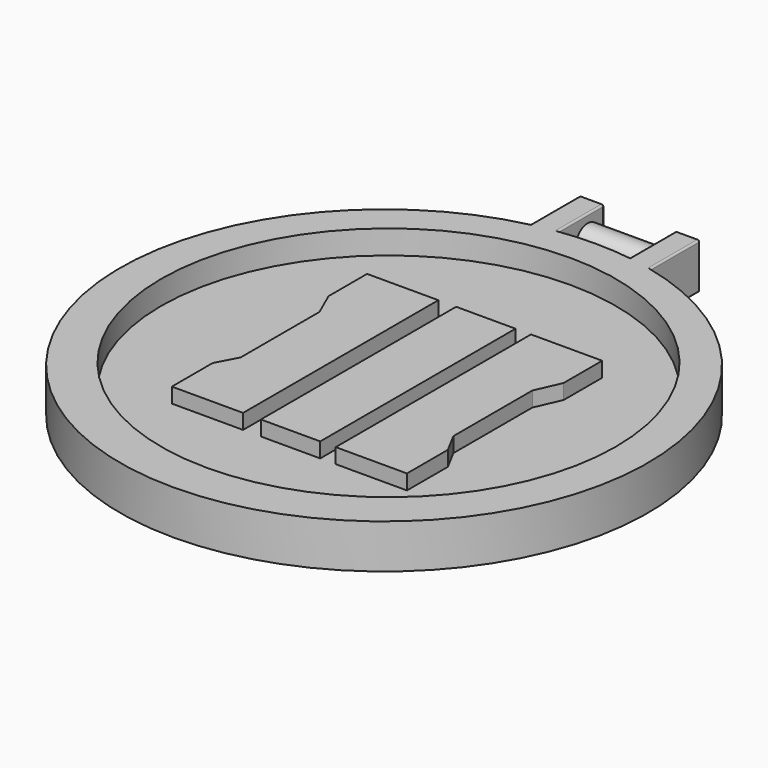
from build123d import *

# Parameters (mm, degrees)
F0_R         = 76.0132265617
F0_R_2       = 65.4635898971
F1_DEPTH     = 12.7
F2_DEPTH     = 10.16
F0_W         = 17.0915899798
F0_H         = 70.289157331
F3_R         = 67.422384844
F4_DEPTH     = 5.842
F5_W         = 6.9010015448
F5_H         = 18.1752619196
F6_DEPTH     = 13.208
F7_T1_DEPTH  = 5.8850015448
F7_T3_DEPTH  = 5.8850015448
F7_T5_DEPTH  = 12.192
F7_T7_DEPTH  = 18.9372619196
F7_S11_W     = 0.508
F7_S11_H     = 0.508
F7_T12_DEPTH = 0.508
F7_S17_W     = 0.508
F7_S17_H     = 0.508
F7_T18_DEPTH = 0.508
F7_S23_W     = 0.508
F7_S23_H     = 0.508
F7_T24_DEPTH = 0.508
F7_S29_W     = 0.508
F7_S29_H     = 0.508
F7_T30_DEPTH = 0.508
F7_S35_W     = 0.508
F7_S35_H     = 0.508
F7_T36_DEPTH = 0.508
F7_S41_W     = 0.508
F7_S41_H     = 0.508
F7_T42_DEPTH = 0.508
F7_S47_W     = 0.508
F7_S47_H     = 0.508
F7_T48_DEPTH = 0.508
F7_S53_W     = 0.508
F7_S53_H     = 0.508
F7_T54_DEPTH = 0.508
F7_T60_DEPTH = 17.6605161867
F7_S61_R     = 76.0132265617
F7_T62_DEPTH = 10
F7_T66_DEPTH = 18.9372619196
F7_S67_R     = 76.0132265617
F7_T68_DEPTH = 11
F7_T72_DEPTH = 17.6605161867
F7_S73_R     = 76.0132265617
F7_T74_DEPTH = 10
F7_T78_DEPTH = 18.9372619196
F7_S79_R     = 76.0132265617
F7_T80_DEPTH = 11
F8_R         = 4.2547927507
F9_DEPTH     = 25.4


# Not quite as in the source:
# - a fillet or chamfer that OpenCascade refuses, or shapes differently, is made with other operations: its cross-section is extruded or revolved along the edge and cut away or added


with BuildPart() as f1:
    # F0 (on Top) → F1 (new body)
    with BuildSketch(Plane.XY):
        Circle(F0_R)
        with Locations((0, 1.6023365315)):
            Circle(F0_R_2, mode=Mode.SUBTRACT)
    extrude(amount=F1_DEPTH)

    # F5 (on face) → F6 (join)
    with BuildSketch(Plane.XY.offset(12.7)):
        with Locations((-13.8136995892, 83.1143693602)):
            Rectangle(F5_W, F5_H)
        with Locations((13.8136995892, 83.1143693602)):
            Rectangle(F5_W, F5_H)
    extrude(amount=-F6_DEPTH)

    # F7: fillet of radius 0.508 on 16 edges, made by hand

    # F7_s2 → F7_t1 (cut)
    with BuildSketch(Plane.YZ.offset(-16.7562003616)):
        with BuildLine():
            ThreePointArc((92.20200032, 12.192), (92.0532105648, 12.5512102448), (91.69400032, 12.7))
            Line((91.69400032, 12.7), (92.20200032, 12.7))
            Line((92.20200032, 12.7), (92.20200032, 12.192))
        make_face()
        with BuildLine():
            ThreePointArc((91.69400032, -0.508), (92.0532105648, -0.3592102448), (92.20200032, 0))
            Line((92.20200032, 0), (92.20200032, -0.508))
            Line((92.20200032, -0.508), (91.69400032, -0.508))
        make_face()
    extrude(amount=F7_T1_DEPTH, mode=Mode.SUBTRACT)

    # F7_s4 → F7_t3 (cut)
    with BuildSketch(Plane.YZ.offset(10.8711988168)):
        with BuildLine():
            ThreePointArc((92.20200032, 12.192), (92.0532105648, 12.5512102448), (91.69400032, 12.7))
            Line((91.69400032, 12.7), (92.20200032, 12.7))
            Line((92.20200032, 12.7), (92.20200032, 12.192))
        make_face()
        with BuildLine():
            ThreePointArc((91.69400032, -0.508), (92.0532105648, -0.3592102448), (92.20200032, 0))
            Line((92.20200032, 0), (92.20200032, -0.508))
            Line((92.20200032, -0.508), (91.69400032, -0.508))
        make_face()
    extrude(amount=F7_T3_DEPTH, mode=Mode.SUBTRACT)

    # F7_s6 → F7_t5 (cut)
    with BuildSketch(Plane.XY):
        with BuildLine():
            ThreePointArc((17.2642003616, 91.69400032), (17.1154106065, 92.0532105648), (16.7562003616, 92.20200032))
            Line((16.7562003616, 92.20200032), (17.2642003616, 92.20200032))
            Line((17.2642003616, 92.20200032), (17.2642003616, 91.69400032))
        make_face()
        with BuildLine():
            ThreePointArc((10.3631988168, 91.69400032), (10.5119885719, 92.0532105648), (10.8711988168, 92.20200032))
            Line((10.8711988168, 92.20200032), (10.3631988168, 92.20200032))
            Line((10.3631988168, 92.20200032), (10.3631988168, 91.69400032))
        make_face()
        with BuildLine():
            ThreePointArc((-16.7562003616, 92.20200032), (-17.1154106065, 92.0532105648), (-17.2642003616, 91.69400032))
            Line((-17.2642003616, 91.69400032), (-17.2642003616, 92.20200032))
            Line((-17.2642003616, 92.20200032), (-16.7562003616, 92.20200032))
        make_face()
        with BuildLine():
            ThreePointArc((-10.3631988168, 91.69400032), (-10.5119885719, 92.0532105648), (-10.8711988168, 92.20200032))
            Line((-10.8711988168, 92.20200032), (-10.3631988168, 92.20200032))
            Line((-10.3631988168, 92.20200032), (-10.3631988168, 91.69400032))
        make_face()
    extrude(amount=F7_T5_DEPTH, mode=Mode.SUBTRACT)

    # F7_s8 → F7_t7 (cut)
    with BuildSketch(Plane.XZ.offset(-91.69400032)):
        with BuildLine():
            ThreePointArc((10.8711988168, -0.508), (10.5119885719, -0.3592102448), (10.3631988168, 0))
            Line((10.3631988168, 0), (10.3631988168, -0.508))
            Line((10.3631988168, -0.508), (10.8711988168, -0.508))
        make_face()
        with BuildLine():
            ThreePointArc((-16.7562003616, -0.508), (-17.1154106065, -0.3592102448), (-17.2642003616, 0))
            Line((-17.2642003616, 0), (-17.2642003616, -0.508))
            Line((-17.2642003616, -0.508), (-16.7562003616, -0.508))
        make_face()
        with BuildLine():
            ThreePointArc((17.2642003616, 0), (17.1154106065, -0.3592102448), (16.7562003616, -0.508))
            Line((16.7562003616, -0.508), (17.2642003616, -0.508))
            Line((17.2642003616, -0.508), (17.2642003616, 0))
        make_face()
        with BuildLine():
            ThreePointArc((-10.3631988168, 0), (-10.5119885719, -0.3592102448), (-10.8711988168, -0.508))
            Line((-10.8711988168, -0.508), (-10.3631988168, -0.508))
            Line((-10.3631988168, -0.508), (-10.3631988168, 0))
        make_face()
    extrude(amount=F7_T7_DEPTH, mode=Mode.SUBTRACT)


with BuildPart() as f2:
    # F0 (on Top) → F2 (new body)
    with BuildSketch(Plane.XY):
        Polygon((-13.3424317464, -34.0763553977), (-13.3424317464, 36.2128019333), (-33.8523387909, 36.2128019333), (-33.8523387909, 22.3258882761), (-30.6476652622, 15.0619633496), (-30.6476652622, -13.3528038859), (-33.8523387909, -19.334860146), (-33.8523387909, -34.0763553977), align=None)
    extrude(amount=F2_DEPTH)


with BuildPart() as f2b:
    # F0 (on Top) → F2, piece 2 (new body)
    with BuildSketch(Plane.XY):
        with Locations((0.3308397718, 1.0682232678)):
            Rectangle(F0_W, F0_H)
    extrude(amount=F2_DEPTH)


with BuildPart() as f2c:
    # F0 (on Top) → F2, piece 3 (new body)
    with BuildSketch(Plane.XY):
        Polygon((33.8523387909, 36.2128019333), (13.3424317464, 36.2128019333), (13.3424317464, -34.0763553977), (33.8523387909, -34.0763553977), (33.8523387909, -19.334860146), (30.6476652622, -13.3528038859), (30.6476652622, 15.0619633496), (33.8523387909, 22.3258882761), align=None)
    extrude(amount=F2_DEPTH)


with BuildPart() as f4:
    # F3 (on Top) → F4 (new body)
    with BuildSketch(Plane.XY):
        Circle(F3_R)
    extrude(amount=F4_DEPTH)


with BuildPart() as f7_tool10:
    # F7_s11 → F7_t12 (new body)
    with BuildSketch(Plane.XZ.offset(-91.69400032)):
        with Locations((-10.6171988168, 12.446)):
            Rectangle(F7_S11_W, F7_S11_H)
    extrude(amount=-F7_T12_DEPTH)

    # F7_s13 → F7_t14 (revolve, cut)
    with BuildSketch(Plane(origin=(-10.8711988168, 91.69400032, 12.192), x_dir=(-0.7071067812, 0, -0.7071067812), z_dir=(0.7071067812, 0, -0.7071067812))):
        with BuildLine():
            ThreePointArc((0, -0.508), (0.508, 0), (0, 0.508))
            Line((0, 0.508), (0, -0.508))
        make_face()
    revolve(axis=Axis((-10.8711988168, 91.69400032, 12.192), (0, 1, 0)), mode=Mode.SUBTRACT)


with BuildPart() as f1_1:
    add(f1.part)

    # F7_t9: cut F7_tool10
    add(f7_tool10.part, mode=Mode.SUBTRACT)


with BuildPart() as f7_tool16:
    # F7_s17 → F7_t18 (new body)
    with BuildSketch(Plane.XZ.offset(-91.69400032)):
        with Locations((-17.0102003616, 12.446)):
            Rectangle(F7_S17_W, F7_S17_H)
    extrude(amount=-F7_T18_DEPTH)

    # F7_s19 → F7_t20 (revolve, cut)
    with BuildSketch(Plane(origin=(-16.7562003616, 91.69400032, 12.192), x_dir=(0.7071067812, 0, -0.7071067812), z_dir=(0.7071067812, 0, 0.7071067812))):
        with BuildLine():
            ThreePointArc((0, -0.508), (0.508, 0), (0, 0.508))
            Line((0, 0.508), (0, -0.508))
        make_face()
    revolve(axis=Axis((-16.7562003616, 91.69400032, 12.192), (0, 1, 0)), mode=Mode.SUBTRACT)


with BuildPart() as f1_2:
    add(f1_1.part)

    # F7_t15: cut F7_tool16
    add(f7_tool16.part, mode=Mode.SUBTRACT)


with BuildPart() as f7_tool22:
    # F7_s23 → F7_t24 (new body)
    with BuildSketch(Plane.XZ.offset(-91.69400032)):
        with Locations((17.0102003616, 12.446)):
            Rectangle(F7_S23_W, F7_S23_H)
    extrude(amount=-F7_T24_DEPTH)

    # F7_s25 → F7_t26 (revolve, cut)
    with BuildSketch(Plane(origin=(16.7562003616, 91.69400032, 12.192), x_dir=(-0.7071067812, 0, -0.7071067812), z_dir=(0.7071067812, 0, -0.7071067812))):
        with BuildLine():
            ThreePointArc((0, -0.508), (0.508, 0), (0, 0.508))
            Line((0, 0.508), (0, -0.508))
        make_face()
    revolve(axis=Axis((16.7562003616, 91.69400032, 12.192), (0, 1, 0)), mode=Mode.SUBTRACT)


with BuildPart() as f1_3:
    add(f1_2.part)

    # F7_t21: cut F7_tool22
    add(f7_tool22.part, mode=Mode.SUBTRACT)


with BuildPart() as f7_tool28:
    # F7_s29 → F7_t30 (new body)
    with BuildSketch(Plane.YZ.offset(10.8711988168)):
        with Locations((91.94800032, 12.446)):
            Rectangle(F7_S29_W, F7_S29_H)
    extrude(amount=-F7_T30_DEPTH)

    # F7_s31 → F7_t32 (revolve, cut)
    with BuildSketch(Plane(origin=(10.8711988168, 91.69400032, 12.192), x_dir=(0, -0.7071067812, -0.7071067812), z_dir=(0, 0.7071067812, -0.7071067812))):
        with BuildLine():
            ThreePointArc((0, -0.508), (0.508, 0), (0, 0.508))
            Line((0, 0.508), (0, -0.508))
        make_face()
    revolve(axis=Axis((10.8711988168, 91.69400032, 12.192), (-1, 0, 0)), mode=Mode.SUBTRACT)


with BuildPart() as f1_4:
    add(f1_3.part)

    # F7_t27: cut F7_tool28
    add(f7_tool28.part, mode=Mode.SUBTRACT)


with BuildPart() as f7_tool34:
    # F7_s35 → F7_t36 (new body)
    with BuildSketch(Plane.YZ.offset(16.7562003616)):
        with Locations((91.94800032, -0.254)):
            Rectangle(F7_S35_W, F7_S35_H)
    extrude(amount=F7_T36_DEPTH)

    # F7_s37 → F7_t38 (revolve, cut)
    with BuildSketch(Plane(origin=(16.7562003616, 91.69400032, 0), x_dir=(0, -0.7071067812, 0.7071067812), z_dir=(0, 0.7071067812, 0.7071067812))):
        with BuildLine():
            ThreePointArc((0, -0.508), (0.508, 0), (0, 0.508))
            Line((0, 0.508), (0, -0.508))
        make_face()
    revolve(axis=Axis((16.7562003616, 91.69400032, 0), (1, 0, 0)), mode=Mode.SUBTRACT)


with BuildPart() as f1_5:
    add(f1_4.part)

    # F7_t33: cut F7_tool34
    add(f7_tool34.part, mode=Mode.SUBTRACT)


with BuildPart() as f7_tool40:
    # F7_s41 → F7_t42 (new body)
    with BuildSketch(Plane.XZ.offset(-91.69400032)):
        with Locations((10.6171988168, -0.254)):
            Rectangle(F7_S41_W, F7_S41_H)
    extrude(amount=-F7_T42_DEPTH)

    # F7_s43 → F7_t44 (revolve, cut)
    with BuildSketch(Plane(origin=(10.8711988168, 91.69400032, 0), x_dir=(0.7071067812, 0, 0.7071067812), z_dir=(-0.7071067812, 0, 0.7071067812))):
        with BuildLine():
            ThreePointArc((0, -0.508), (0.508, 0), (0, 0.508))
            Line((0, 0.508), (0, -0.508))
        make_face()
    revolve(axis=Axis((10.8711988168, 91.69400032, 0), (0, 1, 0)), mode=Mode.SUBTRACT)


with BuildPart() as f1_6:
    add(f1_5.part)

    # F7_t39: cut F7_tool40
    add(f7_tool40.part, mode=Mode.SUBTRACT)


with BuildPart() as f7_tool46:
    # F7_s47 → F7_t48 (new body)
    with BuildSketch(Plane.XZ.offset(-91.69400032)):
        with Locations((-17.0102003616, -0.254)):
            Rectangle(F7_S47_W, F7_S47_H)
    extrude(amount=-F7_T48_DEPTH)

    # F7_s49 → F7_t50 (revolve, cut)
    with BuildSketch(Plane(origin=(-16.7562003616, 91.69400032, 0), x_dir=(0.7071067812, 0, 0.7071067812), z_dir=(-0.7071067812, 0, 0.7071067812))):
        with BuildLine():
            ThreePointArc((0, -0.508), (0.508, 0), (0, 0.508))
            Line((0, 0.508), (0, -0.508))
        make_face()
    revolve(axis=Axis((-16.7562003616, 91.69400032, 0), (0, 1, 0)), mode=Mode.SUBTRACT)


with BuildPart() as f1_7:
    add(f1_6.part)

    # F7_t45: cut F7_tool46
    add(f7_tool46.part, mode=Mode.SUBTRACT)


with BuildPart() as f7_tool52:
    # F7_s53 → F7_t54 (new body)
    with BuildSketch(Plane.XZ.offset(-91.69400032)):
        with Locations((-10.6171988168, -0.254)):
            Rectangle(F7_S53_W, F7_S53_H)
    extrude(amount=-F7_T54_DEPTH)

    # F7_s55 → F7_t56 (revolve, cut)
    with BuildSketch(Plane(origin=(-10.8711988168, 91.69400032, 0), x_dir=(-0.7071067812, 0, 0.7071067812), z_dir=(-0.7071067812, 0, -0.7071067812))):
        with BuildLine():
            ThreePointArc((0, -0.508), (0.508, 0), (0, 0.508))
            Line((0, 0.508), (0, -0.508))
        make_face()
    revolve(axis=Axis((-10.8711988168, 91.69400032, 0), (0, 1, 0)), mode=Mode.SUBTRACT)


with BuildPart() as f1_8:
    add(f1_7.part)

    # F7_t51: cut F7_tool52
    add(f7_tool52.part, mode=Mode.SUBTRACT)


with BuildPart() as f7_tool58:
    # F7_s59 → F7_t60 (new body)
    with BuildSketch(Plane.XZ.offset(-91.69400032)):
        with BuildLine():
            ThreePointArc((10.3631988168, 12.192), (10.5119885719, 12.5512102448), (10.8711988168, 12.7))
            Line((10.8711988168, 12.7), (10.3631988168, 12.7))
            Line((10.3631988168, 12.7), (10.3631988168, 12.192))
        make_face()
    extrude(amount=F7_T60_DEPTH)

    # F7_s61 → F7_t62 (cut, symmetric)
    with BuildSketch(Plane.XY.offset(12.4)):
        Circle(F7_S61_R)
    extrude(amount=F7_T62_DEPTH, both=True, mode=Mode.SUBTRACT)


with BuildPart() as f1_9:
    add(f1_8.part)

    # F7_t57: cut F7_tool58
    add(f7_tool58.part, mode=Mode.SUBTRACT)


with BuildPart() as f7_tool64:
    # F7_s65 → F7_t66 (new body)
    with BuildSketch(Plane.XZ.offset(-72.7567384004)):
        with BuildLine():
            ThreePointArc((17.2642003616, 12.192), (17.1154106065, 12.5512102448), (16.7562003616, 12.7))
            Line((16.7562003616, 12.7), (17.2642003616, 12.7))
            Line((17.2642003616, 12.7), (17.2642003616, 12.192))
        make_face()
    extrude(amount=-F7_T66_DEPTH)

    # F7_s67 → F7_t68 (cut, symmetric)
    with BuildSketch(Plane.XY.offset(12.4)):
        Circle(F7_S67_R)
    extrude(amount=F7_T68_DEPTH, both=True, mode=Mode.SUBTRACT)


with BuildPart() as f1_10:
    add(f1_9.part)

    # F7_t63: cut F7_tool64
    add(f7_tool64.part, mode=Mode.SUBTRACT)


with BuildPart() as f7_tool70:
    # F7_s71 → F7_t72 (new body)
    with BuildSketch(Plane.XZ.offset(-74.0334841333)):
        with BuildLine():
            ThreePointArc((-10.3631988168, 12.192), (-10.5119885719, 12.5512102448), (-10.8711988168, 12.7))
            Line((-10.8711988168, 12.7), (-10.3631988168, 12.7))
            Line((-10.3631988168, 12.7), (-10.3631988168, 12.192))
        make_face()
    extrude(amount=-F7_T72_DEPTH)

    # F7_s73 → F7_t74 (cut, symmetric)
    with BuildSketch(Plane.XY.offset(12.4)):
        Circle(F7_S73_R)
    extrude(amount=F7_T74_DEPTH, both=True, mode=Mode.SUBTRACT)


with BuildPart() as f1_11:
    add(f1_10.part)

    # F7_t69: cut F7_tool70
    add(f7_tool70.part, mode=Mode.SUBTRACT)


with BuildPart() as f7_tool76:
    # F7_s77 → F7_t78 (new body)
    with BuildSketch(Plane.XZ.offset(-91.69400032)):
        with BuildLine():
            ThreePointArc((-16.7562003616, 12.7), (-17.1154106065, 12.5512102448), (-17.2642003616, 12.192))
            Line((-17.2642003616, 12.192), (-17.2642003616, 12.7))
            Line((-17.2642003616, 12.7), (-16.7562003616, 12.7))
        make_face()
    extrude(amount=F7_T78_DEPTH)

    # F7_s79 → F7_t80 (cut, symmetric)
    with BuildSketch(Plane.XY.offset(12.4)):
        Circle(F7_S79_R)
    extrude(amount=F7_T80_DEPTH, both=True, mode=Mode.SUBTRACT)


with BuildPart() as f1_12:
    add(f1_11.part)

    # F7_t75: cut F7_tool76
    add(f7_tool76.part, mode=Mode.SUBTRACT)

    # F8 (on face) → F9 (join)
    with BuildSketch(Plane(origin=(10.3631988168, 0, 0), x_dir=(0, -1, 0), z_dir=(-1, 0, 0))):
        with Locations((-86.2456560135, 6.0460111126)):
            Circle(F8_R)
    extrude(amount=F9_DEPTH)


solid = Compound([f2.part, f2b.part, f2c.part, f4.part, f1_12.part])
